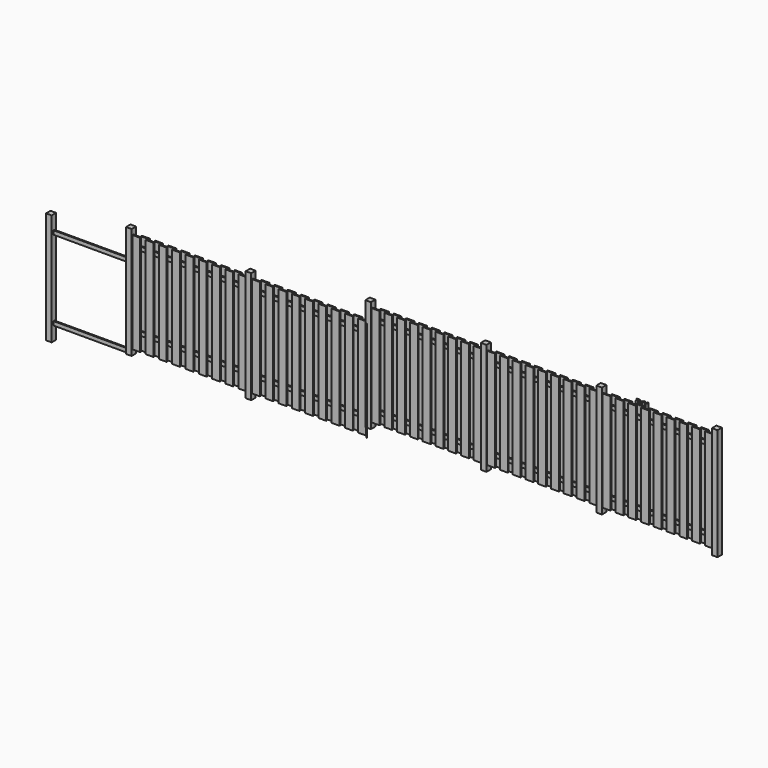
from build123d import *

# Parameters (mm, degrees)
F0_W          = 100
F0_H          = 100
F1_DEPTH      = 2000
F2_DEPTH      = 1760
F2_DEPTH_BACK = 240
F3_DEPTH      = 1510
F3_DEPTH_BACK = 490
F5_START      = -100
F4_W          = 22
F4_H          = 70
F5_DEPTH      = 6100
F6_W          = 22
F6_H          = 70
F7_DEPTH      = 4180
F9_START      = -100
F8_W          = 140
F8_H          = 22
F8_TEXT_SIZE  = 90.4052828749
F9_DEPTH      = 1800
F11_START     = -100
F10_W         = 140
F10_H         = 22
F11_DEPTH     = 1800
F10_W_2       = 2.4971961975
F10_H_2       = 0.4994869232
F13_START     = -10
F12_W         = 22
F12_H         = 70
F13_DEPTH     = 1420


# Not quite as in the source:
# - Text() gives the source's letters only with a copy of the font that has no kerning and outlines rounded to 1/6400 em; it was checked with that copy


with BuildPart() as f1:
    # F0 (on Top) → F1 (new body)
    with BuildSketch(Plane.XY):
        with Locations((-6250, 50)):
            Rectangle(F0_W, F0_H)
    extrude(amount=F1_DEPTH)


with BuildPart() as f1b:
    # F0 (on Top) → F1, piece 2 (new body)
    with BuildSketch(Plane.XY):
        with Locations((-4183, 50)):
            Rectangle(F0_W, F0_H)
    extrude(amount=F1_DEPTH)


with BuildPart() as f1c:
    # F0 (on Top) → F1, piece 3 (new body)
    with BuildSketch(Plane.XY):
        with Locations((-2116.5, 50)):
            Rectangle(F0_W, F0_H)
    extrude(amount=F1_DEPTH)


with BuildPart() as f1d:
    # F0 (on Top) → F1, piece 4 (new body)
    with BuildSketch(Plane.XY):
        with Locations((-50, 50)):
            Rectangle(F0_W, F0_H)
    extrude(amount=F1_DEPTH)


with BuildPart() as f2:
    # F0 (on Top) → F2 (new body, two sides)
    with BuildSketch(Plane.XY) as f2_sk:
        with Locations((-8390, 50)):
            Rectangle(F0_W, F0_H)
    extrude(amount=F2_DEPTH)
    extrude(f2_sk.sketch, amount=-F2_DEPTH_BACK)


with BuildPart() as f2b:
    # F0 (on Top) → F2, piece 2 (new body, two sides)
    with BuildSketch(Plane.XY) as f2_2_sk:
        with Locations((-10530, 50)):
            Rectangle(F0_W, F0_H)
    extrude(amount=F2_DEPTH)
    extrude(f2_2_sk.sketch, amount=-F2_DEPTH_BACK)


with BuildPart() as f3:
    # F0 (on Top) → F3 (new body, two sides)
    with BuildSketch(Plane.XY) as f3_sk:
        with Locations((-11960, 50)):
            Rectangle(F0_W, F0_H)
    extrude(amount=F3_DEPTH)
    extrude(f3_sk.sketch, amount=-F3_DEPTH_BACK)


with BuildPart() as f5:
    # F4 (on face) → F5 (new body)
    with BuildSketch(Plane.YZ.offset(F5_START)):
        with Locations((50, 285)):
            Rectangle(F4_W, F4_H)
    extrude(amount=-F5_DEPTH)


with BuildPart() as f5b:
    # F4 (on face) → F5, piece 2 (new body)
    with BuildSketch(Plane.YZ.offset(F5_START)):
        with Locations((50, 1715)):
            Rectangle(F4_W, F4_H)
    extrude(amount=-F5_DEPTH)


with BuildPart() as f7:
    # F6 (on face) → F7 (new body, through all)
    with BuildSketch(Plane(origin=(-6300, 0, 0), x_dir=(0, -1, 0), z_dir=(-1, 0, 0))):
        with Locations((-50, 1475)):
            Rectangle(F6_W, F6_H)
    extrude(amount=F7_DEPTH)


with BuildPart() as f7b:
    # F6 (on face) → F7, piece 2 (new body, through all)
    with BuildSketch(Plane(origin=(-6300, 0, 0), x_dir=(0, -1, 0), z_dir=(-1, 0, 0))):
        with Locations((-50, 139.7767400742)):
            Rectangle(F6_W, F6_H)
    extrude(amount=F7_DEPTH)


with BuildPart() as f9:
    # F8 (on face) → F9 (new body)
    with BuildSketch(Plane.XY.offset(2000).offset(F9_START)):
        with Locations((-1996.5, 28)):
            Rectangle(F8_W, F8_H)
        with Locations((-1768.2, 28)):
            Rectangle(F8_W, F8_H)
        with Locations((-1539.9, 28)):
            Rectangle(F8_W, F8_H)
        with Locations((-1311.6, 28)):
            Rectangle(F8_W, F8_H)
        with Locations((-1083.3, 28)):
            Rectangle(F8_W, F8_H)
        with Locations((-855, 28)):
            Rectangle(F8_W, F8_H)
        with Locations((-626.7, 28)):
            Rectangle(F8_W, F8_H)
        with Locations((-398.4, 28)):
            Rectangle(F8_W, F8_H)
        with Locations((-170.1, 28)):
            Rectangle(F8_W, F8_H)
        with Locations((-1882.35, 72)):
            Rectangle(F8_W, F8_H)
        with Locations((-1654.05, 72)):
            Rectangle(F8_W, F8_H)
        with Locations((-1425.75, 72)):
            Rectangle(F8_W, F8_H)
        with Locations((-1197.45, 72)):
            Rectangle(F8_W, F8_H)
        with Locations((-969.15, 72)):
            Rectangle(F8_W, F8_H)
        with Locations((-740.85, 72)):
            Rectangle(F8_W, F8_H)
        with Locations((-512.55, 72)):
            Rectangle(F8_W, F8_H)
        with Locations((-284.25, 72)):
            Rectangle(F8_W, F8_H)
        with Locations((-2464.8, 28)):
            Rectangle(F8_W, F8_H)
        with Locations((-2236.5, 28)):
            Rectangle(F8_W, F8_H)
        with Locations((-2578.95, 72)):
            Rectangle(F8_W, F8_H)
        with Locations((-2350.65, 72)):
            Rectangle(F8_W, F8_H)
        with Locations((-2921.4, 28)):
            Rectangle(F8_W, F8_H)
        with Locations((-3263.85, 72)):
            Rectangle(F8_W, F8_H)
        with Locations((-3834.6, 28)):
            Rectangle(F8_W, F8_H)
        with Locations((-2807.25, 72)):
            Rectangle(F8_W, F8_H)
        with Locations((-3720.45, 72)):
            Rectangle(F8_W, F8_H)
        with Locations((-3492.15, 72)):
            Rectangle(F8_W, F8_H)
        with Locations((-3035.55, 72)):
            Rectangle(F8_W, F8_H)
        with Locations((-3948.75, 72)):
            Rectangle(F8_W, F8_H)
        with Locations((-3378, 28)):
            Rectangle(F8_W, F8_H)
        with Locations((-4062.9, 28)):
            Rectangle(F8_W, F8_H)
        with Locations((-3606.3, 28)):
            Rectangle(F8_W, F8_H)
        with Locations((-3149.7, 28)):
            Rectangle(F8_W, F8_H)
        with Locations((-2693.1, 28)):
            Rectangle(F8_W, F8_H)
        with Locations((-4303.1, 28)):
            Rectangle(F8_W, F8_H)
        with Locations((-6129.5, 28)):
            Rectangle(F8_W, F8_H)
        with Locations((-5216.3, 28)):
            Rectangle(F8_W, F8_H)
        with Locations((-4531.4, 28)):
            Rectangle(F8_W, F8_H)
        with Locations((-4417.25, 72)):
            Rectangle(F8_W, F8_H)
        with Locations((-5558.75, 72)):
            Rectangle(F8_W, F8_H)
        with Locations((-4645.55, 72)):
            Rectangle(F8_W, F8_H)
        with Locations((-5330.45, 72)):
            Rectangle(F8_W, F8_H)
        with Locations((-6015.35, 72)):
            Rectangle(F8_W, F8_H)
        with Locations((-5901.2, 28)):
            Rectangle(F8_W, F8_H)
        with Locations((-5444.6, 28)):
            Rectangle(F8_W, F8_H)
        with Locations((-5787.05, 72)):
            Rectangle(F8_W, F8_H)
        with Locations((-4759.7, 28)):
            Rectangle(F8_W, F8_H)
        with Locations((-5102.15, 72)):
            Rectangle(F8_W, F8_H)
        with Locations((-5672.9, 28)):
            Rectangle(F8_W, F8_H)
        with Locations((-4873.85, 72)):
            Rectangle(F8_W, F8_H)
        with Locations((-4988, 28)):
            Rectangle(F8_W, F8_H)
        with Locations((-1596.7940092087, 132.6349526644)):
            Text('Teil 1', F8_TEXT_SIZE, font='Open Sans', text_align=(TextAlign.LEFT, TextAlign.BOTTOM))
    extrude(amount=-F9_DEPTH)


with BuildPart() as f11:
    # F10 (on face) → F11 (new body)
    with BuildSketch(Plane(origin=(0, 0, -240), x_dir=(1, 0, 0), z_dir=(0, 0, -1)).offset(F11_START)):
        with Locations((-6370, -28)):
            Rectangle(F10_W, F10_H)
    extrude(amount=-F11_DEPTH)


with BuildPart() as f11b:
    # F10 (on face) → F11, piece 2 (new body)
    with BuildSketch(Plane(origin=(0, 0, -240), x_dir=(1, 0, 0), z_dir=(0, 0, -1)).offset(F11_START)):
        with Locations((-6246.9713687897, 33.4445089102)):
            Rectangle(F10_W_2, F10_H_2)
    extrude(amount=-F11_DEPTH)


with BuildPart() as f11c:
    # F10 (on face) → F11, piece 3 (new body)
    with BuildSketch(Plane(origin=(0, 0, -240), x_dir=(1, 0, 0), z_dir=(0, 0, -1)).offset(F11_START)):
        with Locations((-6607.5, -28)):
            Rectangle(F10_W, F10_H)
    extrude(amount=-F11_DEPTH)


with BuildPart() as f11d:
    # F10 (on face) → F11, piece 4 (new body)
    with BuildSketch(Plane(origin=(0, 0, -240), x_dir=(1, 0, 0), z_dir=(0, 0, -1)).offset(F11_START)):
        with Locations((-6845, -28)):
            Rectangle(F10_W, F10_H)
    extrude(amount=-F11_DEPTH)


with BuildPart() as f11e:
    # F10 (on face) → F11, piece 5 (new body)
    with BuildSketch(Plane(origin=(0, 0, -240), x_dir=(1, 0, 0), z_dir=(0, 0, -1)).offset(F11_START)):
        with Locations((-7082.5, -28)):
            Rectangle(F10_W, F10_H)
    extrude(amount=-F11_DEPTH)


with BuildPart() as f11f:
    # F10 (on face) → F11, piece 6 (new body)
    with BuildSketch(Plane(origin=(0, 0, -240), x_dir=(1, 0, 0), z_dir=(0, 0, -1)).offset(F11_START)):
        with Locations((-7320, -28)):
            Rectangle(F10_W, F10_H)
    extrude(amount=-F11_DEPTH)


with BuildPart() as f11g:
    # F10 (on face) → F11, piece 7 (new body)
    with BuildSketch(Plane(origin=(0, 0, -240), x_dir=(1, 0, 0), z_dir=(0, 0, -1)).offset(F11_START)):
        with Locations((-7557.5, -28)):
            Rectangle(F10_W, F10_H)
    extrude(amount=-F11_DEPTH)


with BuildPart() as f11h:
    # F10 (on face) → F11, piece 8 (new body)
    with BuildSketch(Plane(origin=(0, 0, -240), x_dir=(1, 0, 0), z_dir=(0, 0, -1)).offset(F11_START)):
        with Locations((-7795, -28)):
            Rectangle(F10_W, F10_H)
    extrude(amount=-F11_DEPTH)


with BuildPart() as f11i:
    # F10 (on face) → F11, piece 9 (new body)
    with BuildSketch(Plane(origin=(0, 0, -240), x_dir=(1, 0, 0), z_dir=(0, 0, -1)).offset(F11_START)):
        with Locations((-8032.5, -28)):
            Rectangle(F10_W, F10_H)
    extrude(amount=-F11_DEPTH)


with BuildPart() as f11j:
    # F10 (on face) → F11, piece 10 (new body)
    with BuildSketch(Plane(origin=(0, 0, -240), x_dir=(1, 0, 0), z_dir=(0, 0, -1)).offset(F11_START)):
        with Locations((-8270, -28)):
            Rectangle(F10_W, F10_H)
    extrude(amount=-F11_DEPTH)


with BuildPart() as f11k:
    # F10 (on face) → F11, piece 11 (new body)
    with BuildSketch(Plane(origin=(0, 0, -240), x_dir=(1, 0, 0), z_dir=(0, 0, -1)).offset(F11_START)):
        with Locations((-6488.75, -72)):
            Rectangle(F10_W, F10_H)
    extrude(amount=-F11_DEPTH)


with BuildPart() as f11l:
    # F10 (on face) → F11, piece 12 (new body)
    with BuildSketch(Plane(origin=(0, 0, -240), x_dir=(1, 0, 0), z_dir=(0, 0, -1)).offset(F11_START)):
        with Locations((-6726.25, -72)):
            Rectangle(F10_W, F10_H)
    extrude(amount=-F11_DEPTH)


with BuildPart() as f11m:
    # F10 (on face) → F11, piece 13 (new body)
    with BuildSketch(Plane(origin=(0, 0, -240), x_dir=(1, 0, 0), z_dir=(0, 0, -1)).offset(F11_START)):
        with Locations((-6963.75, -72)):
            Rectangle(F10_W, F10_H)
    extrude(amount=-F11_DEPTH)


with BuildPart() as f11n:
    # F10 (on face) → F11, piece 14 (new body)
    with BuildSketch(Plane(origin=(0, 0, -240), x_dir=(1, 0, 0), z_dir=(0, 0, -1)).offset(F11_START)):
        with Locations((-7201.25, -72)):
            Rectangle(F10_W, F10_H)
    extrude(amount=-F11_DEPTH)


with BuildPart() as f11o:
    # F10 (on face) → F11, piece 15 (new body)
    with BuildSketch(Plane(origin=(0, 0, -240), x_dir=(1, 0, 0), z_dir=(0, 0, -1)).offset(F11_START)):
        with Locations((-7438.75, -72)):
            Rectangle(F10_W, F10_H)
    extrude(amount=-F11_DEPTH)


with BuildPart() as f11p:
    # F10 (on face) → F11, piece 16 (new body)
    with BuildSketch(Plane(origin=(0, 0, -240), x_dir=(1, 0, 0), z_dir=(0, 0, -1)).offset(F11_START)):
        with Locations((-7676.25, -72)):
            Rectangle(F10_W, F10_H)
    extrude(amount=-F11_DEPTH)


with BuildPart() as f11q:
    # F10 (on face) → F11, piece 17 (new body)
    with BuildSketch(Plane(origin=(0, 0, -240), x_dir=(1, 0, 0), z_dir=(0, 0, -1)).offset(F11_START)):
        with Locations((-7913.75, -72)):
            Rectangle(F10_W, F10_H)
    extrude(amount=-F11_DEPTH)


with BuildPart() as f11r:
    # F10 (on face) → F11, piece 18 (new body)
    with BuildSketch(Plane(origin=(0, 0, -240), x_dir=(1, 0, 0), z_dir=(0, 0, -1)).offset(F11_START)):
        with Locations((-8151.25, -72)):
            Rectangle(F10_W, F10_H)
    extrude(amount=-F11_DEPTH)


with BuildPart() as f11s:
    # F10 (on face) → F11, piece 19 (new body)
    with BuildSketch(Plane(origin=(0, 0, -240), x_dir=(1, 0, 0), z_dir=(0, 0, -1)).offset(F11_START)):
        with Locations((-10410, -28)):
            Rectangle(F10_W, F10_H)
    extrude(amount=-F11_DEPTH)


with BuildPart() as f11t:
    # F10 (on face) → F11, piece 20 (new body)
    with BuildSketch(Plane(origin=(0, 0, -240), x_dir=(1, 0, 0), z_dir=(0, 0, -1)).offset(F11_START)):
        with Locations((-10172.5, -28)):
            Rectangle(F10_W, F10_H)
    extrude(amount=-F11_DEPTH)


with BuildPart() as f11u:
    # F10 (on face) → F11, piece 21 (new body)
    with BuildSketch(Plane(origin=(0, 0, -240), x_dir=(1, 0, 0), z_dir=(0, 0, -1)).offset(F11_START)):
        with Locations((-10053.75, -72)):
            Rectangle(F10_W, F10_H)
    extrude(amount=-F11_DEPTH)


with BuildPart() as f11v:
    # F10 (on face) → F11, piece 22 (new body)
    with BuildSketch(Plane(origin=(0, 0, -240), x_dir=(1, 0, 0), z_dir=(0, 0, -1)).offset(F11_START)):
        with Locations((-10291.25, -72)):
            Rectangle(F10_W, F10_H)
    extrude(amount=-F11_DEPTH)


with BuildPart() as f11w:
    # F10 (on face) → F11, piece 23 (new body)
    with BuildSketch(Plane(origin=(0, 0, -240), x_dir=(1, 0, 0), z_dir=(0, 0, -1)).offset(F11_START)):
        with Locations((-8628.75, -72)):
            Rectangle(F10_W, F10_H)
    extrude(amount=-F11_DEPTH)


with BuildPart() as f11x:
    # F10 (on face) → F11, piece 24 (new body)
    with BuildSketch(Plane(origin=(0, 0, -240), x_dir=(1, 0, 0), z_dir=(0, 0, -1)).offset(F11_START)):
        with Locations((-9578.75, -72)):
            Rectangle(F10_W, F10_H)
    extrude(amount=-F11_DEPTH)


with BuildPart() as f11y:
    # F10 (on face) → F11, piece 25 (new body)
    with BuildSketch(Plane(origin=(0, 0, -240), x_dir=(1, 0, 0), z_dir=(0, 0, -1)).offset(F11_START)):
        with Locations((-9935, -28)):
            Rectangle(F10_W, F10_H)
    extrude(amount=-F11_DEPTH)


with BuildPart() as f11z:
    # F10 (on face) → F11, piece 26 (new body)
    with BuildSketch(Plane(origin=(0, 0, -240), x_dir=(1, 0, 0), z_dir=(0, 0, -1)).offset(F11_START)):
        with Locations((-8747.5, -28)):
            Rectangle(F10_W, F10_H)
    extrude(amount=-F11_DEPTH)


with BuildPart() as f11ba:
    # F10 (on face) → F11, piece 27 (new body)
    with BuildSketch(Plane(origin=(0, 0, -240), x_dir=(1, 0, 0), z_dir=(0, 0, -1)).offset(F11_START)):
        with Locations((-9697.5, -28)):
            Rectangle(F10_W, F10_H)
    extrude(amount=-F11_DEPTH)


with BuildPart() as f11bb:
    # F10 (on face) → F11, piece 28 (new body)
    with BuildSketch(Plane(origin=(0, 0, -240), x_dir=(1, 0, 0), z_dir=(0, 0, -1)).offset(F11_START)):
        with Locations((-9222.5, -28)):
            Rectangle(F10_W, F10_H)
    extrude(amount=-F11_DEPTH)


with BuildPart() as f11bc:
    # F10 (on face) → F11, piece 29 (new body)
    with BuildSketch(Plane(origin=(0, 0, -240), x_dir=(1, 0, 0), z_dir=(0, 0, -1)).offset(F11_START)):
        with Locations((-9103.75, -72)):
            Rectangle(F10_W, F10_H)
    extrude(amount=-F11_DEPTH)


with BuildPart() as f11bd:
    # F10 (on face) → F11, piece 30 (new body)
    with BuildSketch(Plane(origin=(0, 0, -240), x_dir=(1, 0, 0), z_dir=(0, 0, -1)).offset(F11_START)):
        with Locations((-9816.25, -72)):
            Rectangle(F10_W, F10_H)
    extrude(amount=-F11_DEPTH)


with BuildPart() as f11be:
    # F10 (on face) → F11, piece 31 (new body)
    with BuildSketch(Plane(origin=(0, 0, -240), x_dir=(1, 0, 0), z_dir=(0, 0, -1)).offset(F11_START)):
        with Locations((-8866.25, -72)):
            Rectangle(F10_W, F10_H)
    extrude(amount=-F11_DEPTH)


with BuildPart() as f11bf:
    # F10 (on face) → F11, piece 32 (new body)
    with BuildSketch(Plane(origin=(0, 0, -240), x_dir=(1, 0, 0), z_dir=(0, 0, -1)).offset(F11_START)):
        with Locations((-9341.25, -72)):
            Rectangle(F10_W, F10_H)
    extrude(amount=-F11_DEPTH)


with BuildPart() as f11bg:
    # F10 (on face) → F11, piece 33 (new body)
    with BuildSketch(Plane(origin=(0, 0, -240), x_dir=(1, 0, 0), z_dir=(0, 0, -1)).offset(F11_START)):
        with Locations((-8985, -28)):
            Rectangle(F10_W, F10_H)
    extrude(amount=-F11_DEPTH)


with BuildPart() as f11bh:
    # F10 (on face) → F11, piece 34 (new body)
    with BuildSketch(Plane(origin=(0, 0, -240), x_dir=(1, 0, 0), z_dir=(0, 0, -1)).offset(F11_START)):
        with Locations((-8510, -28)):
            Rectangle(F10_W, F10_H)
    extrude(amount=-F11_DEPTH)


with BuildPart() as f11bi:
    # F10 (on face) → F11, piece 35 (new body)
    with BuildSketch(Plane(origin=(0, 0, -240), x_dir=(1, 0, 0), z_dir=(0, 0, -1)).offset(F11_START)):
        with Locations((-9460, -28)):
            Rectangle(F10_W, F10_H)
    extrude(amount=-F11_DEPTH)


with BuildPart() as f13:
    # F12 (on face) → F13 (new body)
    with BuildSketch(Plane(origin=(-12010, 0, 0), x_dir=(0, -1, 0), z_dir=(-1, 0, 0)).offset(F13_START)):
        with Locations((-50, -205)):
            Rectangle(F12_W, F12_H)
    extrude(amount=-F13_DEPTH)


with BuildPart() as f13b:
    # F12 (on face) → F13, piece 2 (new body)
    with BuildSketch(Plane(origin=(-12010, 0, 0), x_dir=(0, -1, 0), z_dir=(-1, 0, 0)).offset(F13_START)):
        with Locations((-50, 1225)):
            Rectangle(F12_W, F12_H)
    extrude(amount=-F13_DEPTH)


solid = Compound([f1.part, f1b.part, f1c.part, f1d.part, f2.part, f2b.part, f3.part, f5.part, f5b.part, f7.part, f7b.part, f9.part, f11.part, f11b.part, f11c.part, f11d.part, f11e.part, f11f.part, f11g.part, f11h.part, f11i.part, f11j.part, f11k.part, f11l.part, f11m.part, f11n.part, f11o.part, f11p.part, f11q.part, f11r.part, f11s.part, f11t.part, f11u.part, f11v.part, f11w.part, f11x.part, f11y.part, f11z.part, f11ba.part, f11bb.part, f11bc.part, f11bd.part, f11be.part, f11bf.part, f11bg.part, f11bh.part, f11bi.part, f13.part, f13b.part])
